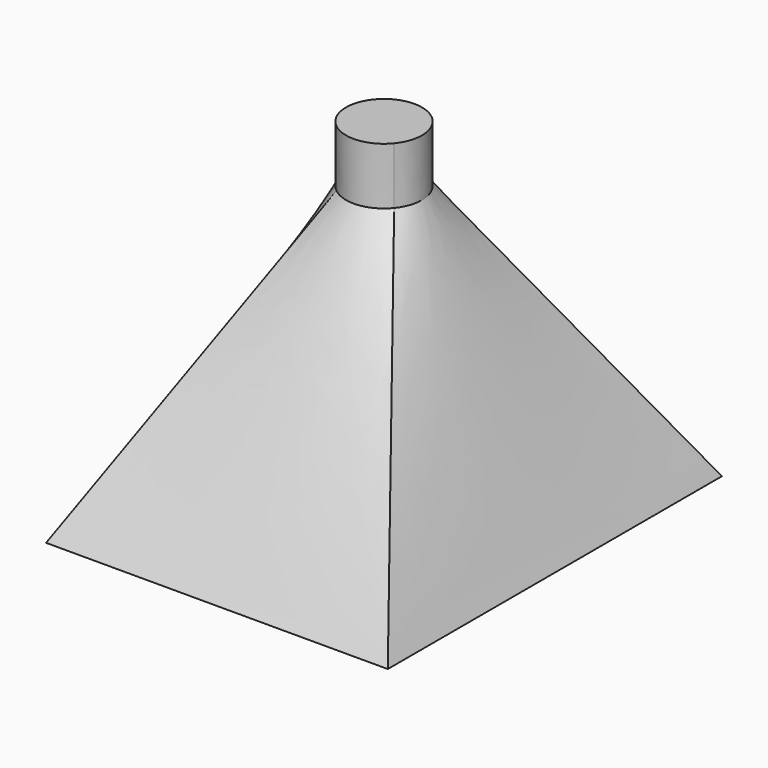
from build123d import *

# Parameters (mm, degrees)
F0_W     = 457.2
F0_H     = 558.8
F4_DEPTH = 76.2


# Not quite as in the source:
# - the arcs of a loft's sections are written as splines that run evenly, so that the points pair up as in the source's solid


with BuildPart() as f3:
    # F0 (on Top) → F3 section 0
    with BuildSketch(Plane.XY):
        with Locations((228.6, 279.4)):
            Rectangle(F0_W, F0_H)
    # F2 (on offset) → F3 section 1
    with BuildSketch(Plane.XY.offset(381)):
        with BuildLine():
            add(Edge.make_bspline(
                [(196.4315202549, 240.0829692005), (199.0048139033, 237.9775471245), (201.7854047693, 236.125618145), (207.6545967757, 232.9997335558), (210.7430527889, 231.7258552398), (217.1092997477, 229.805056205), (220.3869332755, 229.1581829817), (227.0055838864, 228.516284731), (230.3464373104, 228.5212755757), (236.9631405421, 229.1829458989), (240.2388267389, 229.8396090163), (246.599306397, 231.7794202939), (249.6839425829, 233.0625204885), (255.5437690011, 236.205926861), (258.3188143375, 238.066155312), (263.4527976727, 242.2923574354), (265.8116087236, 244.6582266066), (267.9170307995, 247.2315202549)],
                knots=[0, 0, 0, 0, 0.125, 0.125, 0.25, 0.25, 0.375, 0.375, 0.5, 0.5, 0.625, 0.625, 0.75, 0.75, 0.875, 0.875, 1, 1, 1, 1], degree=3))
            add(Edge.make_bspline(
                [(267.9170307995, 247.2315202549), (270.0224528755, 249.8048139033), (271.874381855, 252.5854047693), (275.0002664442, 258.4545967757), (276.2741447602, 261.5430527889), (278.194943795, 267.9092997477), (278.8418170183, 271.1869332755), (279.483715269, 277.8055838864), (279.4787244243, 281.1464373104), (278.8170541011, 287.7631405421), (278.1603909837, 291.0388267389), (276.2205797061, 297.399306397), (274.9374795115, 300.4839425829), (271.794073139, 306.3437690011), (269.933844688, 309.1188143375), (265.7076425646, 314.2527976727), (263.3417733934, 316.6116087236), (260.7684797451, 318.7170307995)],
                knots=[0, 0, 0, 0, 0.125, 0.125, 0.25, 0.25, 0.375, 0.375, 0.5, 0.5, 0.625, 0.625, 0.75, 0.75, 0.875, 0.875, 1, 1, 1, 1], degree=3))
            add(Edge.make_bspline(
                [(260.7684797451, 318.7170307995), (258.1951860967, 320.8224528755), (255.4145952307, 322.674381855), (249.5454032243, 325.8002664442), (246.4569472111, 327.0741447602), (240.0907002523, 328.994943795), (236.8130667245, 329.6418170183), (230.1944161136, 330.283715269), (226.8535626896, 330.2787244243), (220.2368594579, 329.6170541011), (216.9611732611, 328.9603909837), (210.600693603, 327.0205797061), (207.5160574171, 325.7374795115), (201.6562309989, 322.594073139), (198.8811856625, 320.733844688), (193.7472023273, 316.5076425646), (191.3883912764, 314.1417733934), (189.2829692005, 311.5684797451)],
                knots=[0, 0, 0, 0, 0.125, 0.125, 0.25, 0.25, 0.375, 0.375, 0.5, 0.5, 0.625, 0.625, 0.75, 0.75, 0.875, 0.875, 1, 1, 1, 1], degree=3))
            add(Edge.make_bspline(
                [(189.2829692005, 311.5684797451), (187.1775471245, 308.9951860967), (185.325618145, 306.2145952307), (182.1997335558, 300.3454032243), (180.9258552398, 297.2569472111), (179.005056205, 290.8907002523), (178.3581829817, 287.6130667245), (177.716284731, 280.9944161136), (177.7212755757, 277.6535626896), (178.3829458989, 271.0368594579), (179.0396090163, 267.7611732611), (180.9794202939, 261.400693603), (182.2625204885, 258.3160574171), (185.405926861, 252.4562309989), (187.266155312, 249.6811856625), (191.4923574354, 244.5472023273), (193.8582266066, 242.1883912764), (196.4315202549, 240.0829692005)],
                knots=[0, 0, 0, 0, 0.125, 0.125, 0.25, 0.25, 0.375, 0.375, 0.5, 0.5, 0.625, 0.625, 0.75, 0.75, 0.875, 0.875, 1, 1, 1, 1], degree=3))
        make_face()
    loft(ruled=True)

    # F4 (add): a face of the model
    f4_faces = [f3.faces().sort_by_distance(p)[0] for p in [
        (228.6, 279.4, 381),
    ]]
    extrude(f4_faces, amount=F4_DEPTH)


solid = f3.part
